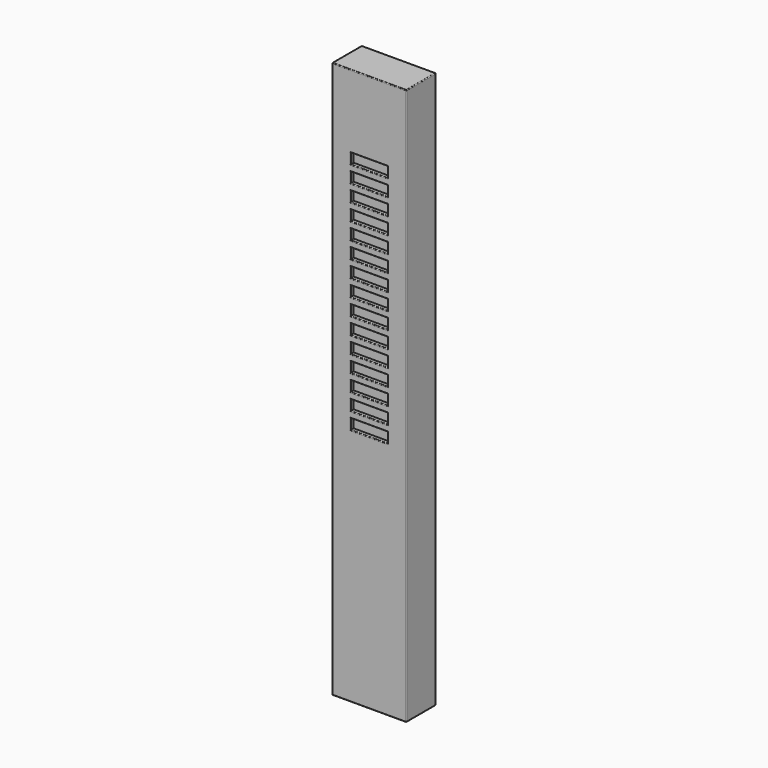
from build123d import *

# Parameters (mm, degrees)
F0_W     = 200
F0_H     = 1500
F0_W_2   = 100
F0_H_2   = 28
F1_DEPTH = 10
F2_W     = 200
F2_H     = 1500
F2_W_2   = 100
F2_H_2   = 28
F3_DEPTH = 6
F5_DEPTH = 68
F6_W     = 168
F6_H     = 1380
F7_DEPTH = 16
F8_R     = 2


# Not quite as in the source:
# - a feature names something its author has since deleted; it is built from what else it names


with BuildPart() as f1:
    # F0 (on Front) → F1 (new body)
    with BuildSketch(Plane.XZ):
        with Locations((0, -2.5)):
            Rectangle(F0_W, F0_H)
        with Locations((0, -93.5)):
            Rectangle(F0_W_2, F0_H_2, mode=Mode.SUBTRACT)
        with Locations((0, -48.5)):
            Rectangle(F0_W_2, F0_H_2, mode=Mode.SUBTRACT)
        with Locations((0, -3.5)):
            Rectangle(F0_W_2, F0_H_2, mode=Mode.SUBTRACT)
        with Locations((0, 41.5)):
            Rectangle(F0_W_2, F0_H_2, mode=Mode.SUBTRACT)
        with Locations((0, 86.5)):
            Rectangle(F0_W_2, F0_H_2, mode=Mode.SUBTRACT)
        with Locations((0, 131.5)):
            Rectangle(F0_W_2, F0_H_2, mode=Mode.SUBTRACT)
        with Locations((0, 176.5)):
            Rectangle(F0_W_2, F0_H_2, mode=Mode.SUBTRACT)
        with Locations((0, 221.5)):
            Rectangle(F0_W_2, F0_H_2, mode=Mode.SUBTRACT)
        with Locations((0, 266.5)):
            Rectangle(F0_W_2, F0_H_2, mode=Mode.SUBTRACT)
        with Locations((0, 311.5)):
            Rectangle(F0_W_2, F0_H_2, mode=Mode.SUBTRACT)
        with Locations((0, 356.5)):
            Rectangle(F0_W_2, F0_H_2, mode=Mode.SUBTRACT)
        with Locations((0, 401.5)):
            Rectangle(F0_W_2, F0_H_2, mode=Mode.SUBTRACT)
        with Locations((0, 446.5)):
            Rectangle(F0_W_2, F0_H_2, mode=Mode.SUBTRACT)
        with Locations((0, 491.5)):
            Rectangle(F0_W_2, F0_H_2, mode=Mode.SUBTRACT)
        with Locations((0, 536.5)):
            Rectangle(F0_W_2, F0_H_2, mode=Mode.SUBTRACT)
    extrude(amount=F1_DEPTH)

    # F2 (on face) → F3 (join)
    with BuildSketch(Plane(origin=(0, 0, 0), x_dir=(-1, 0, 0), z_dir=(0, 1, 0))):
        with Locations((0, -2.5)):
            Rectangle(F2_W, F2_H)
        with Locations((0, -93.5)):
            Rectangle(F2_W_2, F2_H_2, mode=Mode.SUBTRACT)
        with Locations((0, -48.5)):
            Rectangle(F2_W_2, F2_H_2, mode=Mode.SUBTRACT)
        with Locations((0, -3.5)):
            Rectangle(F2_W_2, F2_H_2, mode=Mode.SUBTRACT)
        with Locations((0, 41.5)):
            Rectangle(F2_W_2, F2_H_2, mode=Mode.SUBTRACT)
        with Locations((0, 86.5)):
            Rectangle(F2_W_2, F2_H_2, mode=Mode.SUBTRACT)
        with Locations((0, 131.5)):
            Rectangle(F2_W_2, F2_H_2, mode=Mode.SUBTRACT)
        with Locations((0, 176.5)):
            Rectangle(F2_W_2, F2_H_2, mode=Mode.SUBTRACT)
        with Locations((0, 221.5)):
            Rectangle(F2_W_2, F2_H_2, mode=Mode.SUBTRACT)
        with Locations((0, 266.5)):
            Rectangle(F2_W_2, F2_H_2, mode=Mode.SUBTRACT)
        with Locations((0, 311.5)):
            Rectangle(F2_W_2, F2_H_2, mode=Mode.SUBTRACT)
        with Locations((0, 356.5)):
            Rectangle(F2_W_2, F2_H_2, mode=Mode.SUBTRACT)
        with Locations((0, 401.5)):
            Rectangle(F2_W_2, F2_H_2, mode=Mode.SUBTRACT)
        with Locations((0, 446.5)):
            Rectangle(F2_W_2, F2_H_2, mode=Mode.SUBTRACT)
        with Locations((0, 491.5)):
            Rectangle(F2_W_2, F2_H_2, mode=Mode.SUBTRACT)
        with Locations((0, 536.5)):
            Rectangle(F2_W_2, F2_H_2, mode=Mode.SUBTRACT)
        with Locations((0, -93.5)):
            Rectangle(F2_W_2, F2_H_2)
        with Locations((0, -48.5)):
            Rectangle(F2_W_2, F2_H_2)
        with Locations((0, -3.5)):
            Rectangle(F2_W_2, F2_H_2)
        with Locations((0, 41.5)):
            Rectangle(F2_W_2, F2_H_2)
        with Locations((0, 86.5)):
            Rectangle(F2_W_2, F2_H_2)
        with Locations((0, 131.5)):
            Rectangle(F2_W_2, F2_H_2)
        with Locations((0, 176.5)):
            Rectangle(F2_W_2, F2_H_2)
        with Locations((0, 221.5)):
            Rectangle(F2_W_2, F2_H_2)
        with Locations((0, 266.5)):
            Rectangle(F2_W_2, F2_H_2)
        with Locations((0, 311.5)):
            Rectangle(F2_W_2, F2_H_2)
        with Locations((0, 356.5)):
            Rectangle(F2_W_2, F2_H_2)
        with Locations((0, 401.5)):
            Rectangle(F2_W_2, F2_H_2)
        with Locations((0, 446.5)):
            Rectangle(F2_W_2, F2_H_2)
        with Locations((0, 491.5)):
            Rectangle(F2_W_2, F2_H_2)
        with Locations((0, 536.5)):
            Rectangle(F2_W_2, F2_H_2)
    extrude(amount=F3_DEPTH)

    # F4 (on face) → F5 (join)
    with BuildSketch(Plane(origin=(0, 6, 0), x_dir=(-1, 0, 0), z_dir=(0, 1, 0))):
        Polygon((100, 747.5), (-100, 747.5), (-100, 627.5), (-100, -752.5), (-84, -752.5), (-84, -732.5), (-84, 627.5), (84, 627.5), (84, -732.5), (84, -752.5), (100, -752.5), (100, 727.5), align=None)
    extrude(amount=F5_DEPTH)

    # F6 (on face) → F7 (join)
    with BuildSketch(Plane(origin=(0, 74, 0), x_dir=(-1, 0, 0), z_dir=(0, 1, 0))):
        Polygon((100, 747.5), (-100, 747.5), (-100, -752.5), (-84, -752.5), (-84, 627.5), (84, 627.5), (84, -752.5), (100, -752.5), align=None)
        with Locations((0, -62.5)):
            Rectangle(F6_W, F6_H)
    extrude(amount=F7_DEPTH)

    # F8
    f8_edges = [f1.edges().sort_by_distance(p)[0] for p in [
        (100, 40, -752.5),
        (100, -10, -2.5),
        (100, 40, 747.5),
        (100, 90, -2.5),
        (-100, -10, -2.5),
        (-100, 40, -752.5),
        (-100, 90, -2.5),
        (-100, 40, 747.5),
        (0, -10, 747.5),
        (0, -10, -752.5),
        (0, -10, -107.5),
        (-50, -10, -93.5),
        (0, -10, -79.5),
        (50, -10, -93.5),
        (0, -10, -62.5),
        (-50, -10, -48.5),
        (0, -10, -34.5),
        (50, -10, -48.5),
        (0, -10, -17.5),
        (-50, -10, -3.5),
        (0, -10, 10.5),
        (50, -10, -3.5),
        (0, -10, 27.5),
        (-50, -10, 41.5),
        (0, -10, 55.5),
        (50, -10, 41.5),
        (0, -10, 72.5),
        (-50, -10, 86.5),
        (0, -10, 100.5),
        (50, -10, 86.5),
        (0, -10, 117.5),
        (-50, -10, 131.5),
        (0, -10, 145.5),
        (50, -10, 131.5),
        (0, -10, 162.5),
        (-50, -10, 176.5),
        (0, -10, 190.5),
        (50, -10, 176.5),
        (0, -10, 207.5),
        (-50, -10, 221.5),
        (0, -10, 235.5),
        (50, -10, 221.5),
        (0, -10, 252.5),
        (-50, -10, 266.5),
        (0, -10, 280.5),
        (50, -10, 266.5),
        (0, -10, 297.5),
        (-50, -10, 311.5),
        (0, -10, 325.5),
        (50, -10, 311.5),
        (0, -10, 342.5),
        (-50, -10, 356.5),
        (0, -10, 370.5),
        (50, -10, 356.5),
        (0, -10, 387.5),
        (-50, -10, 401.5),
        (0, -10, 415.5),
        (50, -10, 401.5),
        (0, -10, 432.5),
        (-50, -10, 446.5),
        (0, -10, 460.5),
        (50, -10, 446.5),
        (0, -10, 477.5),
        (-50, -10, 491.5),
        (0, -10, 505.5),
        (50, -10, 491.5),
        (0, -10, 522.5),
        (-50, -10, 536.5),
        (0, -10, 550.5),
        (50, -10, 536.5),
        (0, 90, 747.5),
        (0, 90, -752.5),
    ]]
    fillet(f8_edges, radius=F8_R)


solid = f1.part
